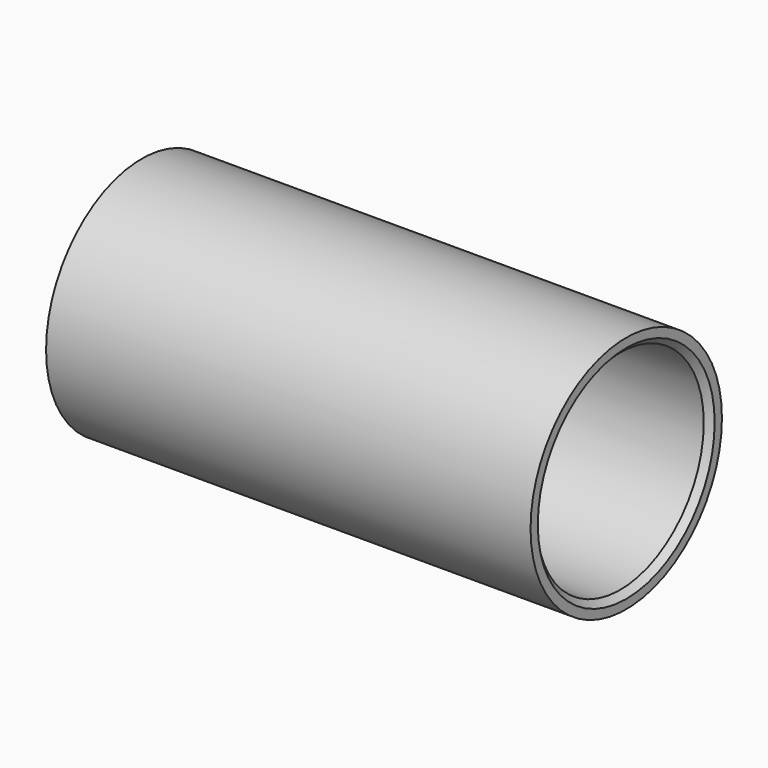
from build123d import *

# Parameters (mm, degrees)
F2_R    = 0.49999
F3_SIZE = 1


# Not quite as in the source:
# - a fillet or chamfer is up to 0.001 mm smaller than in the source, because OpenCascade refuses the exact size


with BuildPart() as f1:
    # F0 (on Top) → F1 (revolve)
    with BuildSketch(Plane.XY):
        Polygon((0, 19.75), (-40, 19.75), (-40, 17.25), (-3.3356409098, 17.25), (-0.5, 16.75), (-0.5, 15.75), (0, 15.75), (0.5, 15.75), (0.5, 16.75), (3.3356409098, 17.25), (40, 17.25), (40, 19.75), align=None)
    revolve(axis=Axis((0, 0, 0), (1, 0, 0)))

    # F2 (radius 0.5 in the source; OpenCascade refuses exactly that, so slightly less here)
    f2_edges = [f1.edges().sort_by_distance(p)[0] for p in [
        (-0.5, -15.75, 0),
        (0.5, -15.75, 0),
    ]]
    fillet(f2_edges, radius=F2_R)

    # F3
    f3_edges = [f1.edges().sort_by_distance(p)[0] for p in [
        (-40, -17.25, 0),
        (40, -17.25, 0),
    ]]
    chamfer(f3_edges, length=F3_SIZE)


solid = f1.part
